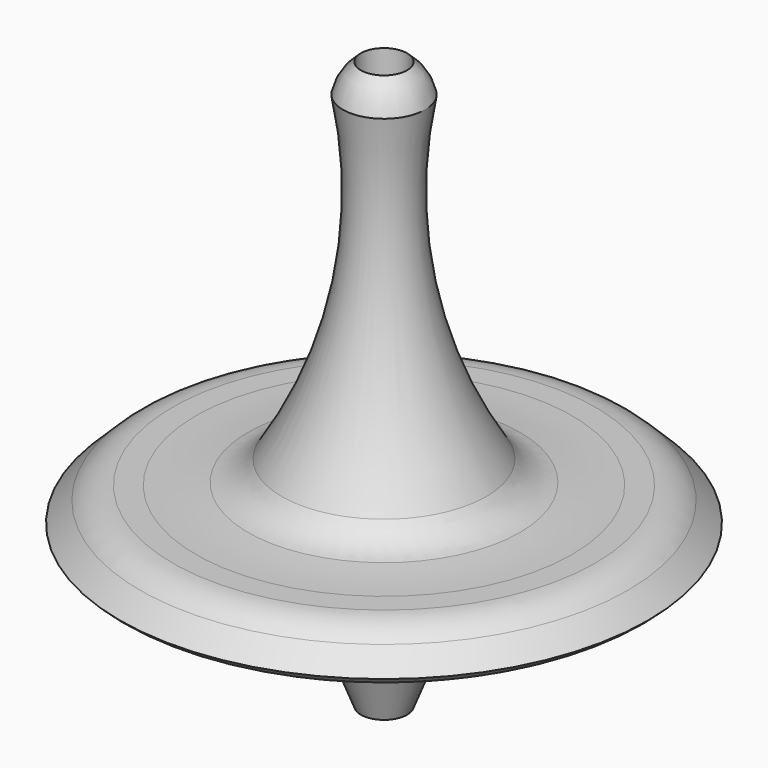
from build123d import *

# Parameters (mm, degrees)
F2_DEPTH = 63.5010001
F3_R     = 5.08
F5_R     = 5.08
F6_R     = 5.08


# Not quite as in the source:
# - a fillet or chamfer that OpenCascade refuses, or shapes differently, is made with other operations: its cross-section is extruded or revolved along the edge and cut away or added


with BuildPart() as f1:
    # F0 (on Front) → F1 (revolve)
    with BuildSketch(Plane.XZ):
        with BuildLine():
            ThreePointArc((4.5341940657, 59.2838630326), (2.9433454488, 62.1191947856), (0, 63.5))
            Line((0, 63.5), (0, 0))
            Line((0, 0), (2.5480911136, 0))
            Line((2.5480911136, 0), (6.6250329837, 10.4471649975))
            Line((6.6250329837, 10.4471649975), (10.9556252941, 16.1543861032))
            Line((10.9556252941, 16.1543861032), (30.48, 16.1543861032))
            Line((30.48, 16.1543861032), (30.4299078499, 21.4240159839))
            Line((30.4299078499, 21.4240159839), (20.699405237, 21.4240159839))
            ThreePointArc((20.699405237, 21.4240159839), (16.6336106625, 21.5337881018), (12.597086859, 22.0329985023))
            ThreePointArc((12.597086859, 22.0329985023), (4.6942529553, 39.8204748482), (4.5341940657, 59.2838630326))
        make_face()
    revolve(axis=Axis((0, 0, 31.75), (0, 0, -1)))

    # F2 (cut, through all): a face of the model
    f2_faces = [f1.faces().sort_by_distance(p)[0] for p in [
        (0, 0, 0),
    ]]
    extrude(f2_faces, amount=-F2_DEPTH, mode=Mode.SUBTRACT)

    # F3
    f3_edges = [f1.edges().sort_by_distance(p)[0] for p in [
        (-10.955625, 0, 16.154386),
        (-30.48, 0, 16.154386),
    ]]
    fillet(f3_edges, radius=F3_R)

    # F4: chamfer of 5.08 on 1 edges, made by hand

    # F4_s1 → F4_t2 (revolve, cut)
    with BuildSketch(Plane.XZ):
        Polygon((30.478195231, 16.3442454843), (25.3499078499, 21.4240159839), (30.4299078499, 21.4240159839), align=None)
    revolve(axis=Axis((0, 0, 21.4240159839), (0, 0, -1)), mode=Mode.SUBTRACT)

    # F5
    f5_edges = [f1.edges().sort_by_distance(p)[0] for p in [
        (-20.699405, 0, 21.424016),
        (-12.597087, 0, 22.032999),
        (16.633611, 0, 21.533788),
    ]]
    fillet(f5_edges, radius=F5_R)

    # F6
    f6_edges = [f1.edges().sort_by_distance(p)[0] for p in [
        (-25.349908, 0, 21.424016),
        (-20.699405, 0, 21.424016),
    ]]
    fillet(f6_edges, radius=F6_R)


solid = f1.part
